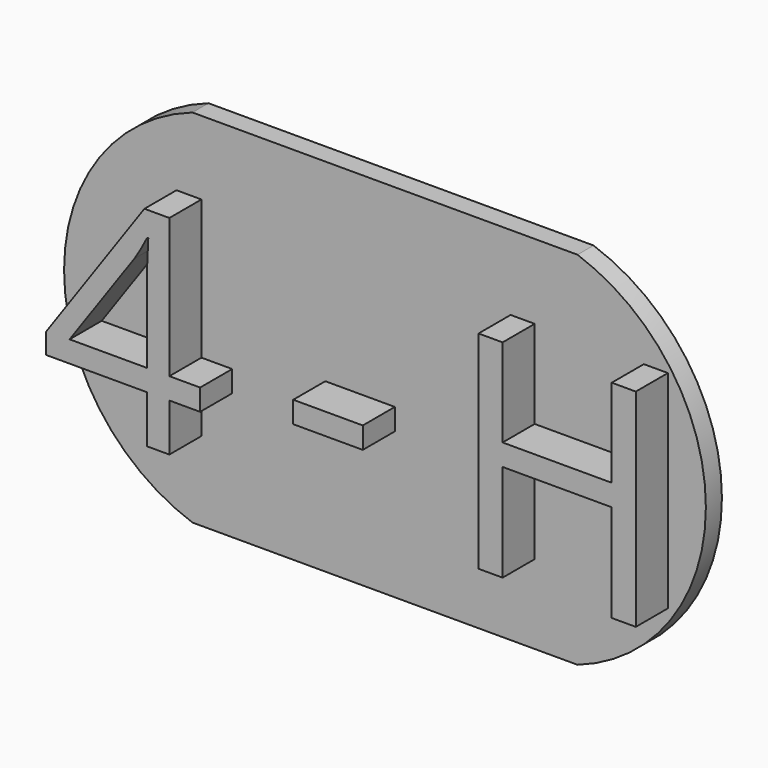
from build123d import *

# Parameters (mm, degrees)
F0_W         = 30.48
F0_H         = 28.575
F1_DEPTH     = 1.5875
F2_TEXT_SIZE = 22.9673563606
F3_DEPTH     = 3.175


# Not quite as in the source:
# - Text() gives the source's letters only with a copy of the font that has no kerning and outlines rounded to 1/6400 em; it was checked with that copy


with BuildPart() as f1:
    # F0 (on Front) → F1 (new body)
    with BuildSketch(Plane.XZ):
        Rectangle(F0_W, F0_H)
        with BuildLine():
            ThreePointArc((15.24, -14.2875), (25.4, 0), (15.24, 14.2875))
            Line((15.24, 14.2875), (15.24, -14.2875))
        make_face()
        with BuildLine():
            Line((-15.24, -14.2875), (-15.24, 14.2875))
            ThreePointArc((-15.24, 14.2875), (-25.4, 0), (-15.24, -14.2875))
        make_face()
    extrude(amount=F1_DEPTH)

    # F2 (on face) → F3 (join)
    with BuildSketch(Plane.XZ.offset(1.5875)):
        with Locations((-24.7644316405, -8.0276979133)):
            Text('4 - H', F2_TEXT_SIZE, font='Open Sans', text_align=(TextAlign.LEFT, TextAlign.BOTTOM))
    extrude(amount=F3_DEPTH)


solid = f1.part
